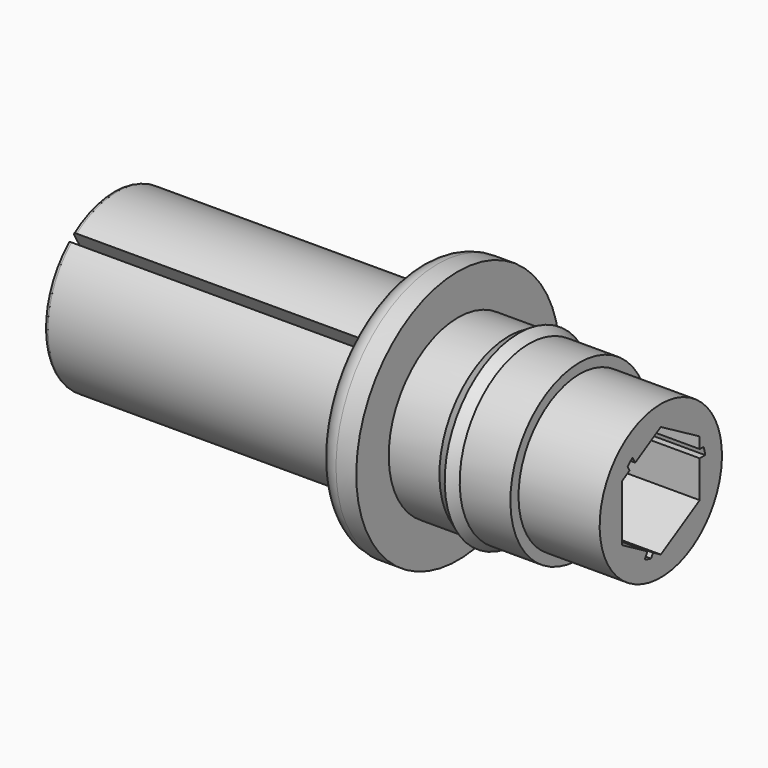
from build123d import *

# Parameters (mm, degrees)
F2_R     = 1
F4_DEPTH = 27
F5_DEPTH = 27
F6_DEPTH = 15
F7_DEPTH = 15
F8_DEPTH = 15
F9_R     = 0.2


with BuildPart() as f1:
    # F0 (on Front) → F1 (revolve)
    with BuildSketch(Plane.XZ):
        Polygon((-9.0454753935, 4.269), (-9.0454753935, 2.769), (17.9545246065, 2.769), (17.9545246065, 3.769), (13.9545246065, 3.769), (13.9545246065, 4.269), (11.4545246065, 4.269), (10.9545246065, 4.569), (10.4545246065, 4.269), (7.9545246065, 4.269), (7.9545246065, 6.269), (5.9545246065, 6.269), (5.9545246065, 4.269), align=None)
    revolve(axis=Axis((2.1683473801, 0, 0), (1, 0, 0)))

    # F2
    f2_edges = [f1.edges().sort_by_distance(p)[0] for p in [
        (5.954525, 0, -6.269),
    ]]
    fillet(f2_edges, radius=F2_R)

    # F3 (on face) → F4 (join)
    with BuildSketch(Plane(origin=(-9.0454753935, 0, 0), x_dir=(0, -1, 0), z_dir=(-1, 0, 0))):
        with BuildLine():
            ThreePointArc((2.769, 0), (2.674648613, 0.7166699359), (2.3980243431, 1.3845))
            Line((2.3980243431, 1.3845), (2.3980243431, -1.3845))
            ThreePointArc((2.3980243431, -1.3845), (2.674648613, -0.7166699359), (2.769, 0))
        make_face()
    extrude(amount=-F4_DEPTH)

    # F3 (on face) → F5 (join)
    with BuildSketch(Plane(origin=(-9.0454753935, 0, 0), x_dir=(0, -1, 0), z_dir=(-1, 0, 0))):
        with BuildLine():
            ThreePointArc((2.769, 0), (2.674648613, 0.7166699359), (2.3980243431, 1.3845))
            Line((2.3980243431, 1.3845), (2.3980243431, -1.3845))
            ThreePointArc((2.3980243431, -1.3845), (2.674648613, -0.7166699359), (2.769, 0))
        make_face()
        with BuildLine():
            Line((1.921710371, 1.6595), (2.3980243431, 1.3845))
            ThreePointArc((2.3980243431, 1.3845), (2.2336171897, 1.6365559111), (2.0428279989, 1.8692818853))
            Line((2.0428279989, 1.8692818853), (1.921710371, 1.6595))
        make_face()
        with BuildLine():
            ThreePointArc((0.9910607425, -2.5855675595), (1.7978084575, -2.1060023148), (2.3980243431, -1.3845))
            Line((2.3980243431, -1.3845), (0.8227241336, -2.294))
            Line((0.8227241336, -2.294), (0.9910607425, -2.5855675595))
        make_face()
        with BuildLine():
            Line((0, 2.769), (1.5753002095, 1.8595))
            Line((1.5753002095, 1.8595), (1.7436368184, 2.1510675595))
            ThreePointArc((1.7436368184, 2.1510675595), (0.9249472763, 2.6099489528), (0, 2.769))
        make_face()
        with BuildLine():
            Line((0.5974316, -2.7037818853), (0.4763139721, -2.494))
            Line((0.4763139721, -2.494), (0, -2.769))
            ThreePointArc((0, -2.769), (0.3004903988, -2.7526471841), (0.5974316, -2.7037818853))
        make_face()
        with BuildLine():
            Line((-2.3980243431, 1.3845), (0, 2.769))
            ThreePointArc((0, 2.769), (-1.3845, 2.3980243431), (-2.3980243431, 1.3845))
        make_face()
        with BuildLine():
            ThreePointArc((-2.3980243431, -1.3845), (-1.3845, -2.3980243431), (0, -2.769))
            Line((0, -2.769), (-2.3980243431, -1.3845))
        make_face()
        with BuildLine():
            Line((-2.3980243431, 0.8345), (-2.3980243431, 1.3845))
            ThreePointArc((-2.3980243431, 1.3845), (-2.5341075885, 1.1160912731), (-2.640259599, 0.8345))
            Line((-2.640259599, 0.8345), (-2.3980243431, 0.8345))
        make_face()
        with BuildLine():
            ThreePointArc((-2.734697561, 0.4345), (-2.7227557338, -0.503946638), (-2.3980243431, -1.3845))
            Line((-2.3980243431, -1.3845), (-2.3980243431, 0.4345))
            Line((-2.3980243431, 0.4345), (-2.734697561, 0.4345))
        make_face()
    extrude(amount=-F5_DEPTH)

    # F3 (on face) → F6 (cut)
    with BuildSketch(Plane(origin=(-9.0454753935, 0, 0), x_dir=(0, -1, 0), z_dir=(-1, 0, 0))):
        with BuildLine():
            ThreePointArc((1.7436368184, 2.1510675595), (1.8984677361, 2.0157334286), (2.0428279989, 1.8692818853))
            Line((2.0428279989, 1.8692818853), (2.8160191704, 3.2084882783))
            ThreePointArc((2.8160191704, 3.2084882783), (2.6608491673, 3.3382993738), (2.4997033736, 3.4606132468))
            Line((2.4997033736, 3.4606132468), (1.7436368184, 2.1510675595))
        make_face()
    extrude(amount=-F6_DEPTH, mode=Mode.SUBTRACT)

    # F3 (on face) → F7 (cut)
    with BuildSketch(Plane(origin=(-9.0454753935, 0, 0), x_dir=(0, -1, 0), z_dir=(-1, 0, 0))):
        with BuildLine():
            Line((1.7471272977, -3.8951132468), (0.9910607425, -2.5855675595))
            ThreePointArc((0.9910607425, -2.5855675595), (0.7964424884, -2.651988002), (0.5974316, -2.7037818853))
            Line((0.5974316, -2.7037818853), (1.3706227715, -4.0429882783))
            ThreePointArc((1.3706227715, -4.0429882783), (1.5606274795, -3.9735126614), (1.7471272977, -3.8951132468))
        make_face()
    extrude(amount=-F7_DEPTH, mode=Mode.SUBTRACT)

    # F3 (on face) → F8 (cut)
    with BuildSketch(Plane(origin=(-9.0454753935, 0, 0), x_dir=(0, -1, 0), z_dir=(-1, 0, 0))):
        with BuildLine():
            Line((-2.640259599, 0.8345), (-4.1866419419, 0.8345))
            ThreePointArc((-4.1866419419, 0.8345), (-4.2214766468, 0.6352132876), (-4.2468306712, 0.4345))
            Line((-4.2468306712, 0.4345), (-2.734697561, 0.4345))
            ThreePointArc((-2.734697561, 0.4345), (-2.6949102244, 0.6362545734), (-2.640259599, 0.8345))
        make_face()
    extrude(amount=-F8_DEPTH, mode=Mode.SUBTRACT)

    # F9
    f9_edges = [f1.edges().sort_by_distance(p)[0] for p in [
        (-9.045475, 1.560627, 3.973513),
        (-9.045475, -4.221477, -0.635213),
        (-9.045475, 2.660849, -3.338299),
        (-9.045475, 2.398024, -0.475),
        (-9.045475, 1.199012, -2.07675),
        (-9.045475, -0.238157, -2.6315),
        (-9.045475, -2.398024, 0),
        (-9.045475, -2.159867, 1.522),
        (-9.045475, 1.199012, 2.07675),
        (-9.045475, -0.78765, 2.31425),
        (-9.045475, -1.610374, -1.83925),
        (-9.045475, 2.398024, 1.1095),
    ]]
    fillet(f9_edges, radius=F9_R)


solid = f1.part
